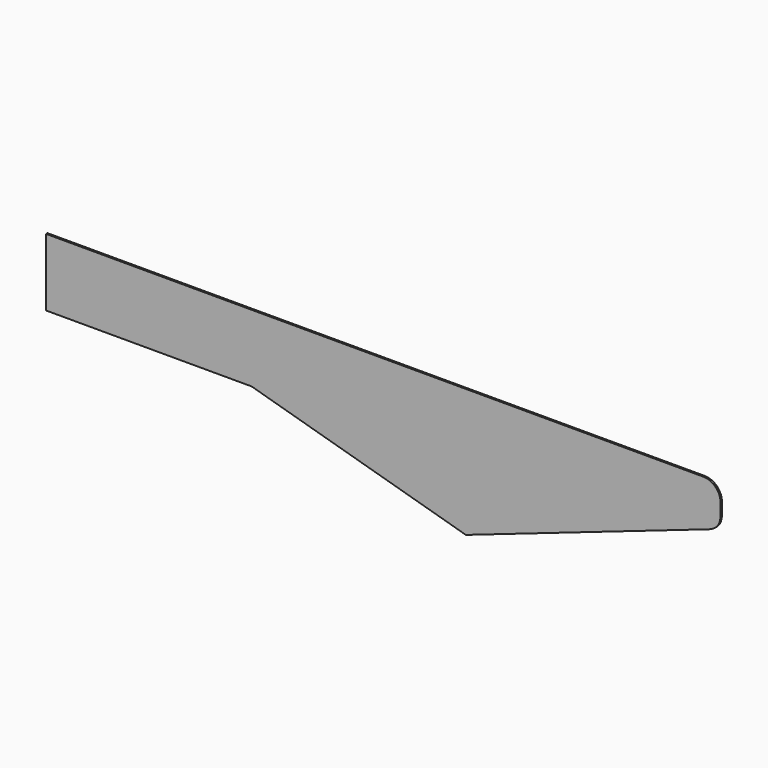
from build123d import *

# Parameters (mm, degrees)
F1_DEPTH    = 2.54
F2_R        = 25.4
F3_T1_DEPTH = 93.0224467373


# Not quite as in the source:
# - a fillet or chamfer that OpenCascade refuses, or shapes differently, is made with other operations: its cross-section is extruded or revolved along the edge and cut away or added


with BuildPart() as f1:
    # F0 (on Front) → F1 (new body)
    with BuildSketch(Plane.XZ):
        Polygon((633.5662589781, 64.4812225811), (-366.4342810219, 64.4812225811), (-366.4342810219, -35.5188314189), (-61.6342810219, -35.5188314189), (255.9216834619, -126.0188282189), (633.5662589781, 4.4813425811), align=None)
    extrude(amount=F1_DEPTH)

    # F2
    f2_edges = [f1.edges().sort_by_distance(p)[0] for p in [
        (633.566259, -1.27, 64.481223),
    ]]
    fillet(f2_edges, radius=F2_R)

    # F3: fillet of radius 25.4 on 1 edges, made by hand

    # F3_s2 → F3_t1 (cut)
    with BuildSketch(Plane.XZ.offset(-45.2412233686)):
        with BuildLine():
            add(Edge.make_bspline(
                [(633.5662589781, 22.5778319285), (633.5662589781, 4.4813425811), (616.4622095682, -1.4291921229)],
                knots=[0, 0, 0, 1, 1, 1], degree=2, weights=[1, 1, 1]))
            Line((616.4622095682, -1.4291921229), (633.5662589781, 4.4813425811))
            Line((633.5662589781, 4.4813425811), (633.5662589781, 22.5778319285))
        make_face()
    extrude(amount=F3_T1_DEPTH, mode=Mode.SUBTRACT)


solid = f1.part
